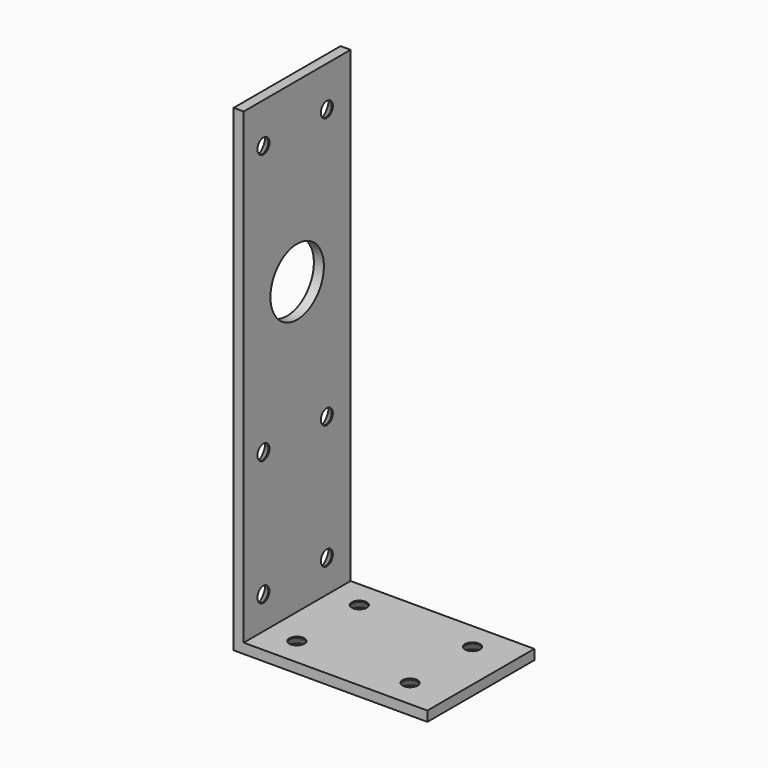
from build123d import *

# Parameters (mm, degrees)
F1_DEPTH       = 40
F3_R           = 10
F4_DEPTH       = 58.001
F6_D           = 4.5
F6_CSINK_D     = 8.96
F6_CSINK_ANGLE = 80
F7_D           = 4.5
F7_CSINK_D     = 8.96
F7_CSINK_ANGLE = 80


# Not quite as in the source:
# - a feature names something its author has since deleted; it is built from what else it names


with BuildPart() as f1:
    # F0 (on Front) → F1 (new body)
    with BuildSketch(Plane.XZ):
        Polygon((3, 143), (0, 143), (0, 0), (58, 0), (58, 3), (3, 3), align=None)
    extrude(amount=F1_DEPTH)

    # F3 (on face) → F4 (cut, through all)
    with BuildSketch(Plane(origin=(0, 0, 0), x_dir=(0, -1, 0), z_dir=(-1, 0, 0))):
        with Locations((20, 90)):
            Circle(F3_R)
    extrude(amount=-F4_DEPTH, mode=Mode.SUBTRACT)

    # F6 (through all)
    with Locations(Plane(origin=(0, 0, 0), x_dir=(0, -1, 0), z_dir=(-1, 0, 0))):
        with Locations((32.6173938811, 50.2130389214), (32.6173938811, 12.7434721217), (8.8956523687, 12.7434721217), (8.8956523687, 49.9434731901), (32.6173938811, 130.9141218662), (8.8956523687, 130.9141218662)):
            CounterSinkHole(F6_D / 2, F6_CSINK_D / 2, counter_sink_angle=F6_CSINK_ANGLE)

    # F7 (through all)
    with Locations(Plane(origin=(0, 0, 0), x_dir=(1, 0, 0), z_dir=(0, 0, -1))):
        with Locations((46.0800911891, 8.2206267661), (12.191168997, 8.2206267661), (12.191168997, 31.5922972435), (46.0800911891, 31.5922972435)):
            CounterSinkHole(F7_D / 2, F7_CSINK_D / 2, counter_sink_angle=F7_CSINK_ANGLE)


solid = f1.part
